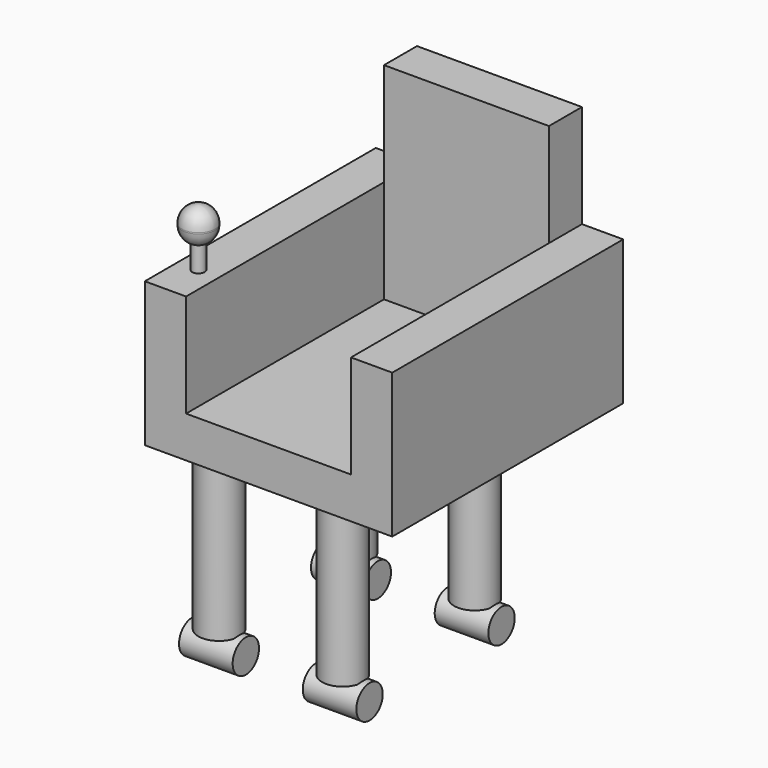
from build123d import *

# Parameters (mm, degrees)
F0_W      = 127
F0_H      = 25.4
F1_DEPTH  = 76.2
F2_R      = 12.7
F3_DEPTH  = 101.6
F5_START  = 20.32
F4_R      = 10.16
F5_DEPTH  = 33.02
F6_START  = 43.18
F5_FACE_R = 10.16
F6_DEPTH  = 33.02
F7_DEPTH  = 25.4
F8_W      = 25.4
F8_H      = 152.4
F9_DEPTH  = 63.5
F10_DEPTH = 25.4
F11_W     = 101.6
F11_H     = 25.4
F12_DEPTH = 127
F13_R     = 3.81
F14_DEPTH = 25.4
F15_R     = 10.16
F16_DEPTH = 10.16


# Not quite as in the source:
# - a fillet or chamfer that OpenCascade refuses, or shapes differently, is made with other operations: its cross-section is extruded or revolved along the edge and cut away or added


with BuildPart() as f1:
    # F0 (on Front) → F1 (new body, symmetric)
    with BuildSketch(Plane.XZ):
        with Locations((-1.2627113611, -2.0410835827)):
            Rectangle(F0_W, F0_H)
    extrude(amount=F1_DEPTH, both=True)

    # F2 (on face) → F3 (join)
    with BuildSketch(Plane(origin=(0, 0, -14.7410835827), x_dir=(1, 0, 0), z_dir=(0, 0, -1))):
        with Locations((-39.3627113611, 50.8)):
            Circle(F2_R)
        with Locations((36.8372886389, 50.8)):
            Circle(F2_R)
        with Locations((36.8372886389, -50.8)):
            Circle(F2_R)
        with Locations((-39.3627113611, -50.8)):
            Circle(F2_R)
    extrude(amount=F3_DEPTH)

    # F4 (on Right) → F5 (join)
    with BuildSketch(Plane.YZ.offset(F5_START)):
        with Locations((-50.8, -125.73)):
            Circle(F4_R)
        with Locations((50.8, -125.73)):
            Circle(F4_R)
    extrude(amount=F5_DEPTH)

    # F5_face (on face) → F6 (join)
    with BuildSketch(Plane(origin=(20.32, 50.8, -125.73), x_dir=(0, 1, 0), z_dir=(-1, 0, 0)).offset(F6_START)):
        Circle(F5_FACE_R)
        with Locations((-101.6, 0)):
            Circle(F5_FACE_R)
    extrude(amount=F6_DEPTH)

    # F7 (add): a face of the model
    f7_faces = [f1.faces().sort_by_distance(p)[0] for p in [
        (62.2372886389, 0, -2.0410835827),
    ]]
    extrude(f7_faces, amount=F7_DEPTH)

    # F8 (on face) → F9 (join)
    with BuildSketch(Plane.XY.offset(10.6589164173)):
        with Locations((74.9372886389, 0)):
            Rectangle(F8_W, F8_H)
        with Locations((-52.0627113611, 0)):
            Rectangle(F8_W, F8_H)
    extrude(amount=F9_DEPTH)

    # F10 (add): a face of the model
    f10_faces = [f1.faces().sort_by_distance(p)[0] for p in [
        (11.4372886389, 76.2, 8.8945760307),
    ]]
    extrude(f10_faces, amount=F10_DEPTH)

    # F11 (on face) → F12 (join)
    with BuildSketch(Plane.XY.offset(10.6589164173)):
        with Locations((11.4372886389, 88.9)):
            Rectangle(F11_W, F11_H)
    extrude(amount=F12_DEPTH)

    # F13 (on face) → F14 (join)
    with BuildSketch(Plane.XY.offset(74.1589164173)):
        with Locations((-52.0627113611, -50.8)):
            Circle(F13_R)
    extrude(amount=F14_DEPTH)

    # F15 (on face) → F16 (join, symmetric)
    with BuildSketch(Plane.XY.offset(99.5589164173)):
        with Locations((-52.0627113611, -50.8)):
            Circle(F15_R)
    extrude(amount=F16_DEPTH, both=True)

    # F17: fillet of radius 10.159746 on 2 edges, made by hand

    # F17_s1 → F17_t2 (revolve, cut)
    with BuildSketch(Plane.XZ.offset(50.8)):
        with BuildLine():
            ThreePointArc((-41.9027113611, 99.5591704173), (-44.8784320693, 106.7431957091), (-52.0624573611, 109.7189164173))
            Line((-52.0624573611, 109.7189164173), (-41.9027113611, 109.7189164173))
            Line((-41.9027113611, 109.7189164173), (-41.9027113611, 99.5591704173))
        make_face()
    revolve(axis=Axis((-52.0627113611, -50.8, 109.7189164173), (0, 0, 1)), mode=Mode.SUBTRACT)

    # F17_s3 → F17_t4 (revolve, cut)
    with BuildSketch(Plane.XZ.offset(50.8)):
        with BuildLine():
            ThreePointArc((-48.2527113611, 89.3989164173), (-43.6384888643, 93.1377755804), (-41.9027113611, 98.8173172476))
            Line((-41.9027113611, 98.8173172476), (-41.9027113611, 89.3989164173))
            Line((-41.9027113611, 89.3989164173), (-48.2527113611, 89.3989164173))
        make_face()
    revolve(axis=Axis((-52.0627113611, -50.8, 89.3989164173), (0, 0, 1)), mode=Mode.SUBTRACT)


solid = f1.part
